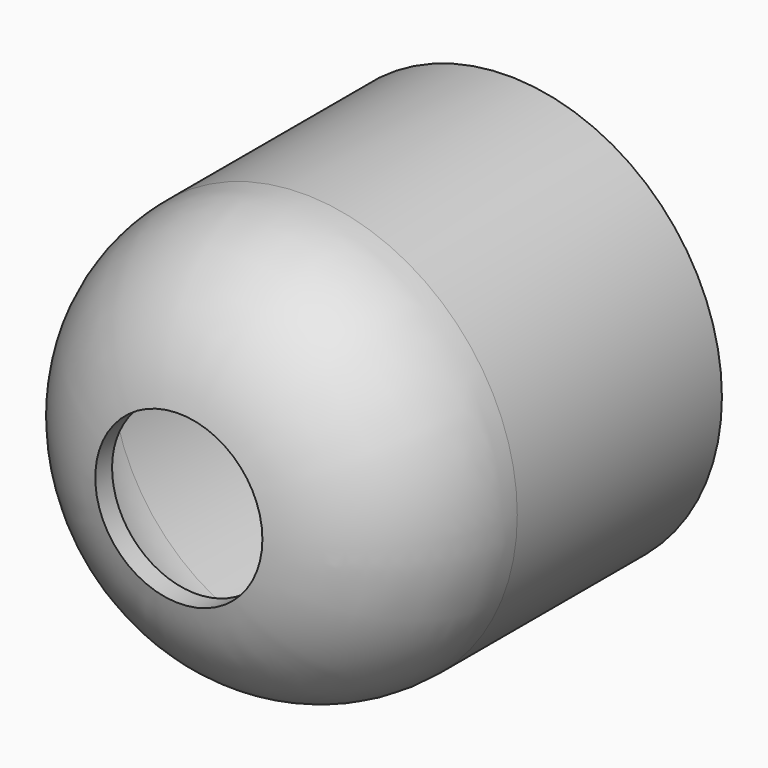
from build123d import *

# Parameters (mm, degrees)
F0_R     = 26.2810947886
F0_R_2   = 10.298862613
F1_DEPTH = 50.8
F3_T     = -2.54


# Not quite as in the source:
# - a fillet or chamfer that OpenCascade refuses, or shapes differently, is made with other operations: its cross-section is extruded or revolved along the edge and cut away or added


with BuildPart() as f1:
    # F0 (on Front) → F1 (new body)
    with BuildSketch(Plane.XZ):
        Circle(F0_R)
        Circle(F0_R_2, mode=Mode.SUBTRACT)
    extrude(amount=F1_DEPTH)

    # F2: fillet of radius 19.622727835 on 1 edges, made by hand

    # F2_s1 → F2_t2 (revolve, cut)
    with BuildSketch(Plane.XY):
        with BuildLine():
            ThreePointArc((26.2810947886, -31.5179295967), (21.7661117091, -44.0402095843), (10.298862613, -50.8))
            Line((10.298862613, -50.8), (26.2810947886, -50.8))
            Line((26.2810947886, -50.8), (26.2810947886, -31.5179295967))
        make_face()
    revolve(axis=Axis((0, -50.8, 0), (0, -1, 0)), mode=Mode.SUBTRACT)

    # F3
    f3_openings = [f1.faces().sort_by_distance(p)[0] for p in [
        (-10.298863, -25.4, 0),
    ]]
    offset(amount=F3_T, openings=f3_openings)


solid = f1.part
